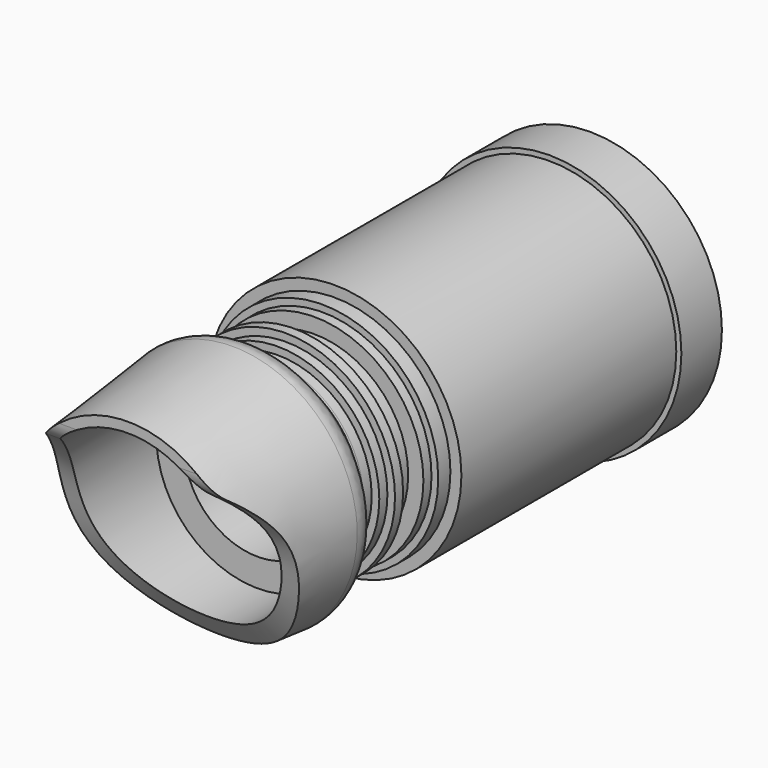
from build123d import *

# Parameters (mm, degrees)
F0_R         = 25
F1_DEPTH     = 53
F2_R         = 26
F3_DEPTH     = 10
F4_R         = 22.8291590373
F5_DEPTH     = 3
F6_R         = 21.5
F7_DEPTH     = 2
F8_R         = 18.5
F9_DEPTH     = 5
F10_R        = 21.5
F11_DEPTH    = 2
F12_R        = 20
F13_DEPTH    = 2
F14_R        = 18.5
F15_DEPTH    = 2
F16_R        = 25
F17_DEPTH    = 35
F18_R        = 20
F19_DEPTH    = 32
F20_S5_R     = 18.5
F20_T6_DEPTH = 37
F22_R        = 5
F25_DEPTH    = 52.3
F26_T1_DEPTH = 15.5791600382
F26_T3_DEPTH = 15.5791600382
F27_R        = 14.5
F28_DEPTH    = 128


# Not quite as in the source:
# - a fillet or chamfer that OpenCascade refuses, or shapes differently, is made with other operations: its cross-section is extruded or revolved along the edge and cut away or added


with BuildPart() as f1:
    # F0 (on Front) → F1 (new body)
    with BuildSketch(Plane.XZ):
        Circle(F0_R)
    extrude(amount=F1_DEPTH)

    # F2 (on face) → F3 (join)
    with BuildSketch(Plane(origin=(0, 0, 0), x_dir=(-1, 0, 0), z_dir=(0, 1, 0))):
        Circle(F2_R)
    extrude(amount=F3_DEPTH)

    # F4 (on face) → F5 (join)
    with BuildSketch(Plane.XZ.offset(53)):
        Circle(F4_R)
    extrude(amount=F5_DEPTH)

    # F6 (on face) → F7 (join)
    with BuildSketch(Plane.XZ.offset(56)):
        Circle(F6_R)
    extrude(amount=F7_DEPTH)

    # F8 (on face) → F9 (join)
    with BuildSketch(Plane.XZ.offset(58)):
        Circle(F8_R)
    extrude(amount=F9_DEPTH)

    # F10 (on face) → F11 (join)
    with BuildSketch(Plane.XZ.offset(63)):
        Circle(F10_R)
    extrude(amount=F11_DEPTH)

    # F12 (on face) → F13 (join)
    with BuildSketch(Plane.XZ.offset(65)):
        Circle(F12_R)
    extrude(amount=F13_DEPTH)

    # F14 (on face) → F15 (join)
    with BuildSketch(Plane.XZ.offset(67)):
        Circle(F14_R)
    extrude(amount=F15_DEPTH)

    # F16 (on face) → F17 (join)
    with BuildSketch(Plane.XZ.offset(69)):
        Circle(F16_R)
    extrude(amount=F17_DEPTH)

    # F18 (on face) → F19 (cut)
    with BuildSketch(Plane.XZ.offset(104)):
        Circle(F18_R)
    extrude(amount=-F19_DEPTH, mode=Mode.SUBTRACT)

    # F20: chamfer of 7 on 1 edges, made by hand


with BuildPart() as f20_tool2:
    # F20_s3 → F20_t4 (revolve)
    with BuildSketch(Plane.XY):
        Polygon((25, -76), (18, -69), (25, -69), align=None)
    revolve(axis=Axis((0, -69, 0), (0, -1, 0)))

    # F20_s5 → F20_t6 (cut, symmetric)
    with BuildSketch(Plane.XZ.offset(72.5)):
        Circle(F20_S5_R)
    extrude(amount=F20_T6_DEPTH, both=True, mode=Mode.SUBTRACT)


with BuildPart() as f1_1:
    add(f1.part)

    # F20_t1: cut F20_tool2
    add(f20_tool2.part, mode=Mode.SUBTRACT)

    # F21: chamfer of 3 x 30 on 1 edges, made by hand

    # F21_s1 → F21_t2 (revolve, cut)
    with BuildSketch(Plane.XY):
        Polygon((25, -74), (22, -104), (25, -104), align=None)
    revolve(axis=Axis((0, -104, 0), (0, -1, 0)), mode=Mode.SUBTRACT)

    # F22
    f22_edges = [f1_1.edges().sort_by_distance(p)[0] for p in [
        (-24.818182, -75.818182, 0),
    ]]
    fillet(f22_edges, radius=F22_R)

    # F24 (on offset) → F25 (cut)
    with BuildSketch(Plane.YZ.offset(26.9)):
        with BuildLine():
            Line((-78, -31.0485586524), (-78, -28.3997934312))
            add(Edge.make_bspline(
                [(-78, -28.3997934312), (-98.6184179783, -3.1667915173), (-82.4469923973, 1.2942913454), (-107.4011772871, 17.0474909246)],
                knots=[0, 0, 0, 0, 54.1284110351, 54.1284110351, 54.1284110351, 54.1284110351], degree=3))
            Line((-107.4011772871, 17.0474909246), (-107.4011772871, -31.0485586524))
            Line((-107.4011772871, -31.0485586524), (-78, -31.0485586524))
        make_face()
    extrude(amount=-F25_DEPTH, mode=Mode.SUBTRACT)

    # F26: fillet of radius 5 on 2 edges, made by hand

    # F26_s2 → F26_t1 (cut)
    with BuildSketch(Plane.YZ.offset(7.0799043749)):
        with BuildLine():
            ThreePointArc((-102.0117387885, 13.3536507945), (-103.4757188766, 15.1160616448), (-104.0004, 17.346317106))
            Line((-104.0004, 17.346317106), (-104.50064, 17.346317106))
            ThreePointArc((-104.50064, 17.346317106), (-104.50024, 16.0708587935), (-104.50024, 14.795400481))
            Line((-104.50024, 14.795400481), (-104.286297169, 14.3851883546))
            ThreePointArc((-104.286297169, 14.3851883546), (-103.2925012303, 13.6788063197), (-102.3131126673, 12.9543841634))
            Line((-102.3131126673, 12.9543841634), (-102.0117387885, 13.3536507945))
        make_face()
    extrude(amount=F26_T1_DEPTH, mode=Mode.SUBTRACT)

    # F26_s4 → F26_t3 (cut)
    with BuildSketch(Plane.YZ.offset(-22.6590644131)):
        with BuildLine():
            ThreePointArc((-102.0117387885, 13.3536507945), (-103.4757188766, 15.1160616448), (-104.0004, 17.346317106))
            Line((-104.0004, 17.346317106), (-104.50064, 17.346317106))
            ThreePointArc((-104.50064, 17.346317106), (-104.50024, 16.0708587935), (-104.50024, 14.795400481))
            Line((-104.50024, 14.795400481), (-104.286297169, 14.3851883546))
            ThreePointArc((-104.286297169, 14.3851883546), (-103.2925012303, 13.6788063197), (-102.3131126673, 12.9543841634))
            Line((-102.3131126673, 12.9543841634), (-102.0117387885, 13.3536507945))
        make_face()
    extrude(amount=F26_T3_DEPTH, mode=Mode.SUBTRACT)

    # F27 (on face) → F28 (cut)
    with BuildSketch(Plane(origin=(0, 10, 0), x_dir=(-1, 0, 0), z_dir=(0, 1, 0))):
        Circle(F27_R)
    extrude(amount=-F28_DEPTH, mode=Mode.SUBTRACT)


solid = f1_1.part
